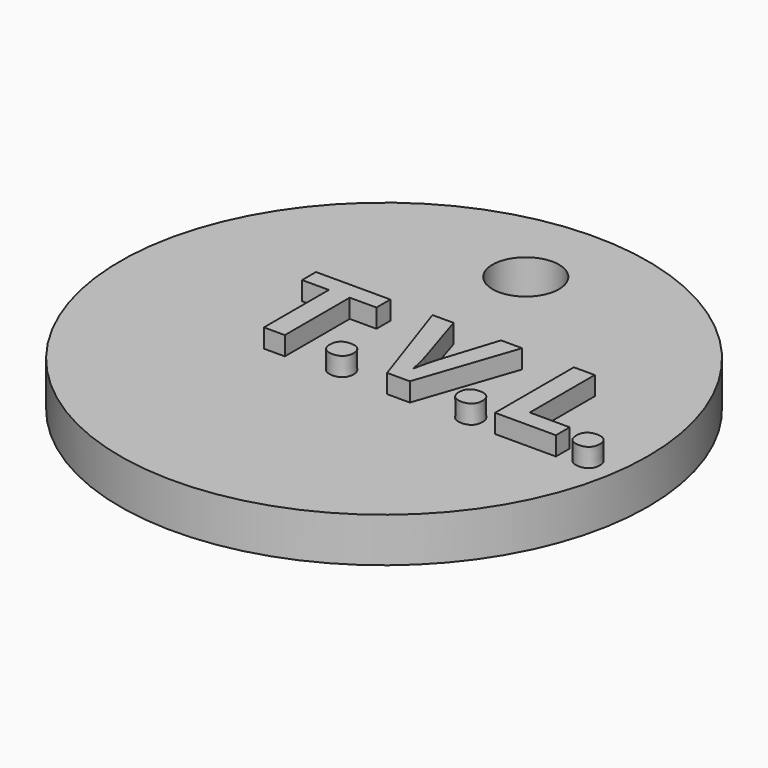
from build123d import *

# Parameters (mm, degrees)
F0_R         = 28.6344541381
F0_R_2       = 3.6087479261
F1_DEPTH     = 4.826
F2_TEXT_SIZE = 14.9685210393
F3_DEPTH     = 6.858


# Not quite as in the source:
# - Text() gives the source's letters only with a copy of the font that has no kerning and outlines rounded to 1/6400 em; it was checked with that copy


with BuildPart() as f1:
    # F0 (on Top) → F1 (new body)
    with BuildSketch(Plane.XY):
        Circle(F0_R)
        with Locations((0, 19.2117728293)):
            Circle(F0_R_2, mode=Mode.SUBTRACT)
    extrude(amount=F1_DEPTH)

    # F2 (on Top) → F3 (join)
    with BuildSketch(Plane.XY):
        with Locations((-12.3002193868, -4.9200877547)):
            Text('T.V.L.', F2_TEXT_SIZE, font='Open Sans', font_style=FontStyle.BOLD, text_align=(TextAlign.LEFT, TextAlign.BOTTOM))
    extrude(amount=F3_DEPTH)


solid = f1.part
